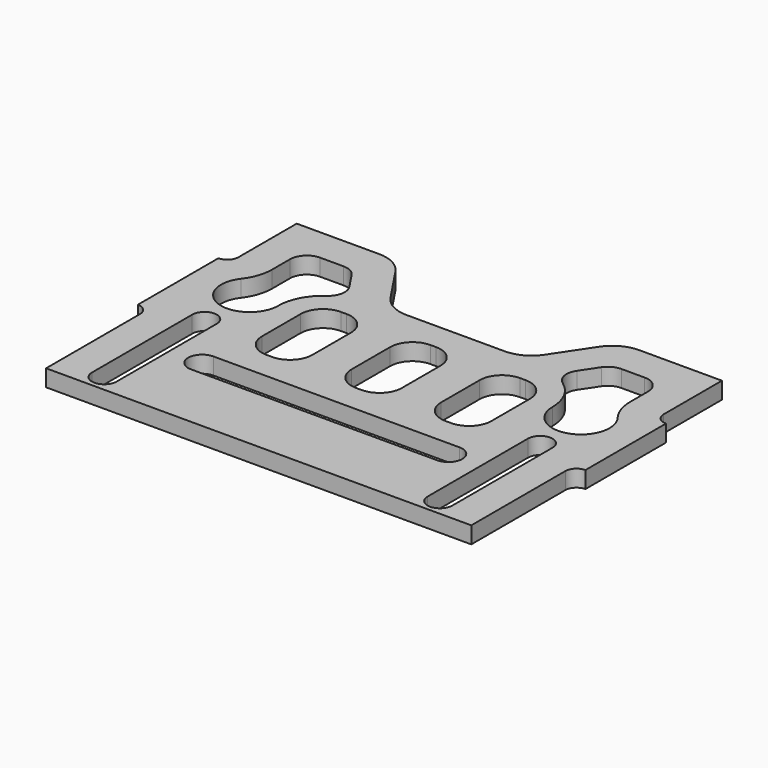
from build123d import *

# Parameters (mm, degrees)
F1_DEPTH = 1.5


# Not quite as in the source:
# - ends of sketch curves that miss each other by under 0.0002 mm in the source are joined


with BuildPart() as f1:
    # F0 (on Top) → F1 (new body)
    with BuildSketch(Plane.XY):
        with BuildLine():
            ThreePointArc((20, 6.5), (19.2928932188, 6.7928932188), (19, 7.5))
            Line((19, 7.5), (19, 14))
            Line((19, 14), (11.605551, 14))
            ThreePointArc((11.605551, 14), (10.1899773457, 13.6450238617), (9.1094002708, 12.6641008194))
            Line((9.1094002708, 12.6641008194), (6.890599, 9.3359))
            ThreePointArc((6.890599, 9.3359), (5.8100220211, 8.3549763346), (4.394448, 8))
            Line((4.394448, 8), (-4.394449, 8))
            ThreePointArc((-4.394449, 8), (-5.8100230211, 8.3549763346), (-6.8906001907, 9.3358998729))
            Line((-6.8906001907, 9.3358998729), (-9.109401, 12.664101))
            ThreePointArc((-9.109401, 12.664101), (-10.1899783457, 13.6450238617), (-11.605552, 14))
            Line((-11.605552, 14), (-19, 14))
            Line((-19, 14), (-19, 7.5))
            ThreePointArc((-19, 7.5), (-19.2928932188, 6.7928932188), (-20, 6.5))
            Line((-20, 6.5), (-20, -2.5))
            ThreePointArc((-20, -2.5), (-19.2928932188, -2.7928932188), (-19, -3.5))
            Line((-19, -3.5), (-19, -14))
            Line((-19, -14), (19, -14))
            Line((19, -14), (19, -3.5))
            ThreePointArc((19, -3.5), (19.2928932188, -2.7928932188), (20, -2.5))
            Line((20, -2.5), (20, 6.5))
        make_face()
        with BuildLine():
            ThreePointArc((-13.9, -12.498995), (-15, -13.598995), (-16.1, -12.498995))
            Line((-16.1, -12.498995), (-16.1, -1.300086))
            ThreePointArc((-16.1, -1.300086), (-15, -0.200086), (-13.9, -1.300086))
            Line((-13.9, -1.300086), (-13.9, -12.498995))
        make_face(mode=Mode.SUBTRACT)
        with BuildLine():
            ThreePointArc((-11, -7.808873), (-12.25, -6.558873), (-11, -5.308873))
            Line((-11, -5.308873), (11, -5.308873))
            ThreePointArc((11, -5.308873), (12.25, -6.558873), (11, -7.808873))
            Line((11, -7.808873), (-11, -7.808873))
        make_face(mode=Mode.SUBTRACT)
        with BuildLine():
            ThreePointArc((16.1, -12.498995), (15, -13.598995), (13.9, -12.498995))
            Line((13.9, -12.498995), (13.9, -1.300086))
            ThreePointArc((13.9, -1.300086), (15, -0.200086), (16.1, -1.300086))
            Line((16.1, -1.300086), (16.1, -12.498995))
        make_face(mode=Mode.SUBTRACT)
        with BuildLine():
            ThreePointArc((-12.25, 3.5), (-15.6295091101, 1.0805038434), (-16.8308317088, 5.0594317757))
            ThreePointArc((-16.8308317088, 5.0594317757), (-16.2134004171, 6.2109446874), (-16, 7.5))
            Line((-16, 7.5), (-16, 9.5))
            ThreePointArc((-16, 9.5), (-15.5606601718, 10.5606601718), (-14.5, 11))
            Line((-14.5, 11), (-12.408327, 11))
            ThreePointArc((-12.408327, 11), (-11.7005404785, 10.8225120945), (-11.16025202, 10.3320509866))
            Line((-11.16025202, 10.3320509866), (-10.161512, 8.83394))
            ThreePointArc((-10.161512, 8.83394), (-9.935298233, 7.7253531463), (-10.5478817855, 6.7741016944))
            ThreePointArc((-10.5478817855, 6.7741016944), (-11.7990510276, 5.3450573983), (-12.25, 3.5))
        make_face(mode=Mode.SUBTRACT)
        with BuildLine():
            Line((-5.75, 3.5), (-5.75, -0.808873))
            ThreePointArc((-5.75, -0.808873), (-6.3357864376, -2.2230865624), (-7.75, -2.808873))
            Line((-7.75, -2.808873), (-8.25, -2.808873))
            ThreePointArc((-8.25, -2.808873), (-9.6642135624, -2.2230865624), (-10.25, -0.808873))
            Line((-10.25, -0.808873), (-10.25, 3.5))
            ThreePointArc((-10.25, 3.5), (-9.6642135624, 4.9142135624), (-8.25, 5.5))
            Line((-8.25, 5.5), (-7.75, 5.5))
            ThreePointArc((-7.75, 5.5), (-6.3357864376, 4.9142135624), (-5.75, 3.5))
        make_face(mode=Mode.SUBTRACT)
        with BuildLine():
            Line((2.25, 3.5), (2.25, -0.808873))
            ThreePointArc((2.25, -0.808873), (1.6642135624, -2.2230865624), (0.25, -2.808873))
            Line((0.25, -2.808873), (-0.25, -2.808873))
            ThreePointArc((-0.25, -2.808873), (-1.6642135624, -2.2230865624), (-2.25, -0.808873))
            Line((-2.25, -0.808873), (-2.25, 3.5))
            ThreePointArc((-2.25, 3.5), (-1.6642135624, 4.9142135624), (-0.25, 5.5))
            Line((-0.25, 5.5), (0.25, 5.5))
            ThreePointArc((0.25, 5.5), (1.6642135624, 4.9142135624), (2.25, 3.5))
        make_face(mode=Mode.SUBTRACT)
        with BuildLine():
            Line((10.25, 3.5), (10.25, -0.808873))
            ThreePointArc((10.25, -0.808873), (9.6642135624, -2.2230865624), (8.25, -2.808873))
            Line((8.25, -2.808873), (7.75, -2.808873))
            ThreePointArc((7.75, -2.808873), (6.3357864376, -2.2230865624), (5.75, -0.808873))
            Line((5.75, -0.808873), (5.75, 3.5))
            ThreePointArc((5.75, 3.5), (6.3357864376, 4.9142135624), (7.75, 5.5))
            Line((7.75, 5.5), (8.25, 5.5))
            ThreePointArc((8.25, 5.5), (9.6642135624, 4.9142135624), (10.25, 3.5))
        make_face(mode=Mode.SUBTRACT)
        with BuildLine():
            ThreePointArc((16.8308313365, 5.0594322592), (15.6295093989, 1.0805039417), (12.25, 3.5))
            ThreePointArc((12.25, 3.5), (11.7990508389, 5.3450577615), (10.5478809284, 6.774101898))
            ThreePointArc((10.5478809284, 6.774101898), (9.9352982087, 7.7253532759), (10.1615112508, 8.8339398328))
            Line((10.1615112508, 8.8339398328), (11.160251, 10.332051))
            ThreePointArc((11.160251, 10.332051), (11.700540234, 10.8225119636), (12.408327, 11))
            Line((12.408327, 11), (14.5, 11))
            ThreePointArc((14.5, 11), (15.5606601718, 10.5606601718), (16, 9.5))
            Line((16, 9.5), (16, 7.5))
            ThreePointArc((16, 7.5), (16.2134003188, 6.2109449762), (16.8308313365, 5.0594322592))
        make_face(mode=Mode.SUBTRACT)
    extrude(amount=F1_DEPTH)


solid = f1.part
